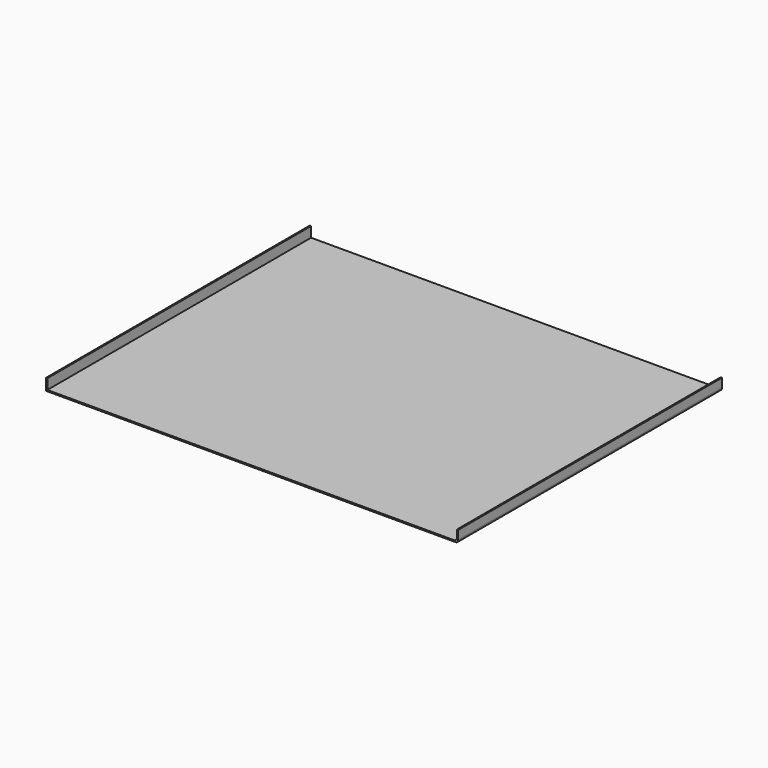
from build123d import *

# Parameters (mm, degrees)
F0_W     = 508
F0_H     = 1.5875
F1_DEPTH = 406.4
F4_DEPTH = 406.4
F5_DEPTH = 406.4
F6_DEPTH = 406.401


# Not quite as in the source:
# - a feature of the source that left no trace in its solid (it failed there, or was rolled back) is left out


with BuildPart() as f1:
    # F0 (on Front) → F1 (new body)
    with BuildSketch(Plane.XZ):
        with Locations((254, 0.79375)):
            Rectangle(F0_W, F0_H)
    extrude(amount=F1_DEPTH)

    # F2 (on face) → F6 (cut, through all)
    with BuildSketch(Plane.XZ.offset(406.4)):
        with BuildLine():
            ThreePointArc((507.6565132189, 1.5875), (506.8812439632, 0.6176396397), (505.8041214943, 0))
            Line((505.8041214943, 0), (508, 0))
            Line((508, 0), (508, 1.5875))
            Line((508, 1.5875), (507.6565132189, 1.5875))
        make_face()
        with BuildLine():
            Line((508, 3.6682041828), (508, 2.6142150412))
            ThreePointArc((508, 2.6142150412), (508.0420476883, 3.141209612), (508, 3.6682041828))
        make_face()
    extrude(amount=-F6_DEPTH, mode=Mode.SUBTRACT)


with BuildPart() as f4:
    # F2 (on face) → F4 (new body)
    with BuildSketch(Plane.XZ.offset(406.4)):
        Polygon((0, 9.3688843772), (0, 1.5875), (1.6079572961, 1.5875), (1.6079572961, 14.2875), (0, 14.2875), (0, 9.9055850878), align=None)
    extrude(amount=-F4_DEPTH)


with BuildPart() as f4b:
    # F2 (on face) → F4, piece 2 (new body)
    with BuildSketch(Plane.XZ.offset(406.4)):
        with BuildLine():
            Line((506.4125, 14.2875), (506.4125, 4.4695332181))
            Line((506.4125, 4.4695332181), (506.4125, 1.5875))
            Line((506.4125, 1.5875), (507.6565132189, 1.5875))
            ThreePointArc((507.6565132189, 1.5875), (507.870344829, 2.0867769369), (508, 2.6142150412))
            Line((508, 2.6142150412), (508, 3.6682041828))
            Line((508, 3.6682041828), (508, 14.2875))
            Line((508, 14.2875), (506.4125, 14.2875))
        make_face()
        with BuildLine():
            Line((508, 3.6682041828), (508, 2.6142150412))
            ThreePointArc((508, 2.6142150412), (508.0420476883, 3.141209612), (508, 3.6682041828))
        make_face()
    extrude(amount=-F4_DEPTH)


with BuildPart() as f5:
    # F2 (on face) → F5 (new body)
    with BuildSketch(Plane.XZ.offset(406.4)):
        with BuildLine():
            ThreePointArc((506.4125, 4.4695332181), (505.364992625, 2.8316639404), (503.8710235621, 1.5875))
            Line((503.8710235621, 1.5875), (506.4125, 1.5875))
            Line((506.4125, 1.5875), (506.4125, 4.4695332181))
        make_face()
    extrude(amount=-F5_DEPTH)


solid = Compound([f1.part, f4.part, f4b.part, f5.part])
